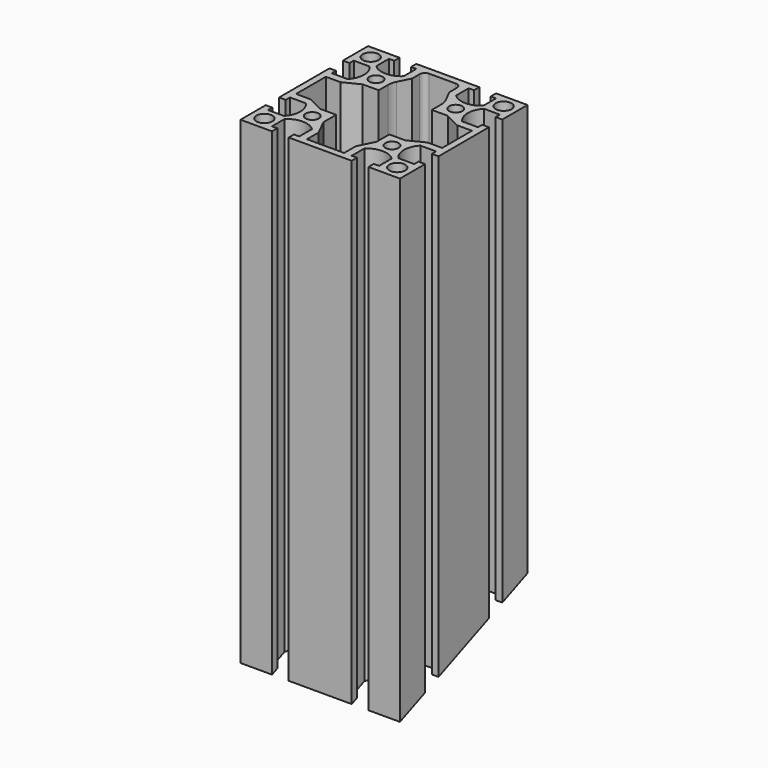
from build123d import *

# Parameters (mm, degrees)
F0_R          = 3
F0_R_2        = 2.5
F1_DEPTH      = 180
F2_R          = 2
F3_R          = 7
F6_DEPTH      = 30
F6_DEPTH_BACK = 30


# Not quite as in the source:
# - a feature names something its author has since deleted; it is built from what else it names


with BuildPart() as f1:
    # F0 (on Top) → F1 (new body)
    with BuildSketch(Plane.XY):
        with BuildLine():
            Line((18.15, -30), (30, -30))
            Line((30, -30), (30, -18.15))
            Line((30, -18.15), (27.5, -18.15))
            Line((27.5, -18.15), (27.5, -20.15))
            Line((27.5, -20.15), (21.5477069044, -20.15))
            ThreePointArc((21.5477069044, -20.15), (19.5, -15), (21.5477069044, -9.85))
            Line((21.5477069044, -9.85), (27.5, -9.85))
            Line((27.5, -9.85), (27.5, -11.85))
            Line((27.5, -11.85), (30, -11.85))
            Line((30, -11.85), (30, 11.85))
            Line((30, 11.85), (27.5, 11.85))
            Line((27.5, 11.85), (27.5, 9.85))
            Line((27.5, 9.85), (21.5477069044, 9.85))
            ThreePointArc((21.5477069044, 9.85), (19.5, 15), (21.5477069044, 20.15))
            Line((21.5477069044, 20.15), (27.5, 20.15))
            Line((27.5, 20.15), (27.5, 18.15))
            Line((27.5, 18.15), (30, 18.15))
            Line((30, 18.15), (30, 30))
            Line((30, 30), (18.15, 30))
            Line((18.15, 30), (18.15, 27.5))
            Line((18.15, 27.5), (20.15, 27.5))
            Line((20.15, 27.5), (20.15, 21.5477069044))
            ThreePointArc((20.15, 21.5477069044), (15, 19.5), (9.85, 21.5477069044))
            Line((9.85, 21.5477069044), (9.85, 27.5))
            Line((9.85, 27.5), (11.85, 27.5))
            Line((11.85, 27.5), (11.85, 30))
            Line((11.85, 30), (-11.85, 30))
            Line((-11.85, 30), (-11.85, 27.5))
            Line((-11.85, 27.5), (-9.85, 27.5))
            Line((-9.85, 27.5), (-9.85, 21.5477069044))
            ThreePointArc((-9.85, 21.5477069044), (-15, 19.5), (-20.15, 21.5477069044))
            Line((-20.15, 21.5477069044), (-20.15, 27.5))
            Line((-20.15, 27.5), (-18.15, 27.5))
            Line((-18.15, 27.5), (-18.15, 30))
            Line((-18.15, 30), (-30, 30))
            Line((-30, 30), (-30, 18.15))
            Line((-30, 18.15), (-27.5, 18.15))
            Line((-27.5, 18.15), (-27.5, 20.15))
            Line((-27.5, 20.15), (-21.5477069044, 20.15))
            ThreePointArc((-21.5477069044, 20.15), (-19.5, 15), (-21.5477069044, 9.85))
            Line((-21.5477069044, 9.85), (-27.5, 9.85))
            Line((-27.5, 9.85), (-27.5, 11.85))
            Line((-27.5, 11.85), (-30, 11.85))
            Line((-30, 11.85), (-30, -11.85))
            Line((-30, -11.85), (-27.5, -11.85))
            Line((-27.5, -11.85), (-27.5, -9.85))
            Line((-27.5, -9.85), (-21.5477069044, -9.85))
            ThreePointArc((-21.5477069044, -9.85), (-19.5, -15), (-21.5477069044, -20.15))
            Line((-21.5477069044, -20.15), (-27.5, -20.15))
            Line((-27.5, -20.15), (-27.5, -18.15))
            Line((-27.5, -18.15), (-30, -18.15))
            Line((-30, -18.15), (-30, -30))
            Line((-30, -30), (-18.15, -30))
            Line((-18.15, -30), (-18.15, -27.5))
            Line((-18.15, -27.5), (-20.15, -27.5))
            Line((-20.15, -27.5), (-20.15, -21.5477069044))
            ThreePointArc((-20.15, -21.5477069044), (-15, -19.5), (-9.85, -21.5477069044))
            Line((-9.85, -21.5477069044), (-9.85, -27.5))
            Line((-9.85, -27.5), (-11.85, -27.5))
            Line((-11.85, -27.5), (-11.85, -30))
            Line((-11.85, -30), (11.85, -30))
            Line((11.85, -30), (11.85, -27.5))
            Line((11.85, -27.5), (9.85, -27.5))
            Line((9.85, -27.5), (9.85, -21.5477069044))
            ThreePointArc((9.85, -21.5477069044), (15, -19.5), (20.15, -21.5477069044))
            Line((20.15, -21.5477069044), (20.15, -27.5))
            Line((20.15, -27.5), (18.15, -27.5))
            Line((18.15, -27.5), (18.15, -30))
        make_face()
        with Locations((-25, -25)):
            Circle(F0_R, mode=Mode.SUBTRACT)
        with Locations((-15, -15)):
            Circle(F0_R_2, mode=Mode.SUBTRACT)
        with Locations((25, -25)):
            Circle(F0_R, mode=Mode.SUBTRACT)
        with Locations((15, -15)):
            Circle(F0_R_2, mode=Mode.SUBTRACT)
        with Locations((-25, 25)):
            Circle(F0_R, mode=Mode.SUBTRACT)
        with Locations((-15, 15)):
            Circle(F0_R_2, mode=Mode.SUBTRACT)
        Polygon((-7, 22), (-7, 27.5), (0, 27.5), (7, 27.5), (7, 22), (10, 16), (10, 10), (16, 10), (22, 7), (27.5, 7), (27.5, 0), (27.5, -7), (22, -7), (16, -10), (10, -10), (10, -16), (7, -22), (7, -27.5), (0, -27.5), (-7, -27.5), (-7, -22), (-10, -16), (-10, -10), (-16, -10), (-22, -7), (-27.5, -7), (-27.5, 0), (-27.5, 7), (-22, 7), (-16, 10), (-10, 10), (-10, 16), align=None, mode=Mode.SUBTRACT)
        with Locations((15, 15)):
            Circle(F0_R_2, mode=Mode.SUBTRACT)
        with Locations((25, 25)):
            Circle(F0_R, mode=Mode.SUBTRACT)
    extrude(amount=F1_DEPTH)

    # F2
    f2_edges = [f1.edges().sort_by_distance(p)[0] for p in [
        (-7, 27.5, 90),
        (7, 27.5, 90),
    ]]
    fillet(f2_edges, radius=F2_R)

    # F3
    f3_edges = [f1.edges().sort_by_distance(p)[0] for p in [
        (-10, 16, 90),
        (10, 16, 90),
    ]]
    fillet(f3_edges, radius=F3_R)

    # F5 (on Right) → F6 (cut, two sides)
    with BuildSketch(Plane.YZ) as f6_sk:
        Polygon((189.0217391842, -31.0070544887), (145.9840988475, 72.8950005046), (-30, 0), (13.0376403367, -103.9020549933), align=None)
    extrude(amount=-F6_DEPTH, mode=Mode.SUBTRACT)
    extrude(f6_sk.sketch, amount=F6_DEPTH_BACK, mode=Mode.SUBTRACT)


solid = f1.part
